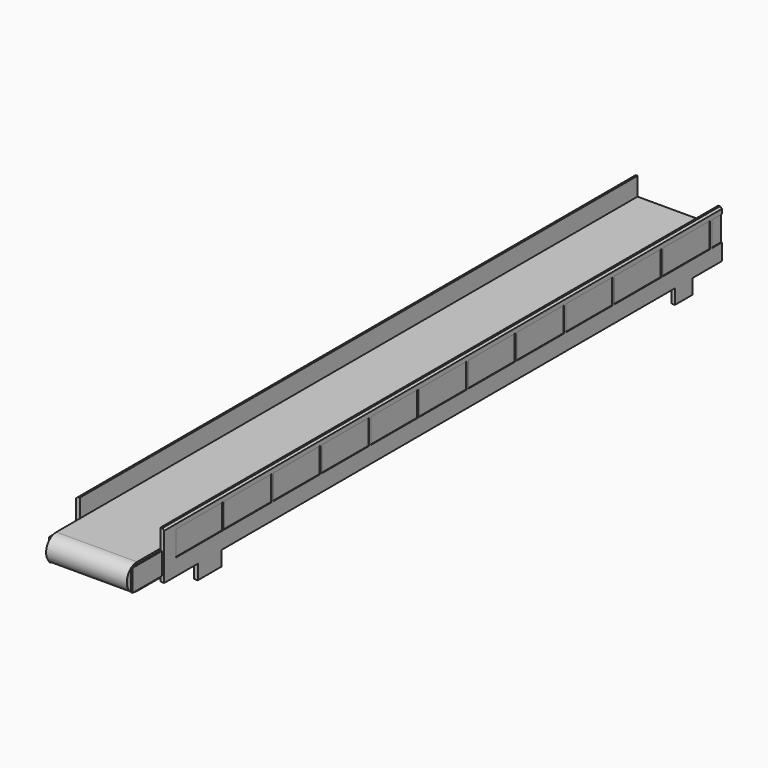
from build123d import *

# Parameters (mm, degrees)
F1_R          = 150
F2_DEPTH      = 1100
F4_DEPTH      = 1100
F6_START      = -400
F6_DEPTH      = 12000
F7_W          = 20
F7_H          = 300
F8_DEPTH      = 500
F8_DEPTH_BACK = 12500
F9_W          = 800
F9_H          = 340
F10_DEPTH     = 10
F11_W         = 800
F11_H         = 340
F12_DEPTH     = 10
F13_W         = 50
F13_H         = 400
F14_DEPTH     = 200
F15_W         = 1814.6319389343
F15_H         = 1127.1775364876
F16_DEPTH     = 3000
F17_W         = 50
F17_H         = 300
F18_DEPTH     = 200


with BuildPart() as f2:
    # F1 (on Right) → F2 (new body)
    with BuildSketch(Plane.YZ):
        Circle(F1_R)
    extrude(amount=F2_DEPTH)


with BuildPart() as f2b:
    # F1 (on Right) → F2, piece 2 (new body)
    with BuildSketch(Plane.YZ):
        with Locations((12700, 0)):
            Circle(F1_R)
    extrude(amount=F2_DEPTH)


with BuildPart() as f4:
    # F3 (on face) → F4 (new body)
    with BuildSketch(Plane.YZ.offset(1100)):
        with BuildLine():
            ThreePointArc((0, -175), (123.7436867076, -123.7436867076), (175, 0))
            ThreePointArc((175, 0), (123.7436867076, 123.7436867076), (0, 175))
            Line((0, 175), (0, -175))
        make_face()
        with BuildLine():
            ThreePointArc((0, 175), (123.7436867076, 123.7436867076), (175, 0))
            ThreePointArc((175, 0), (123.7436867076, -123.7436867076), (0, -175))
            Line((0, -175), (12700, -175))
            ThreePointArc((12700, -175), (12525, 0), (12700, 175))
            Line((12700, 175), (0, 175))
        make_face()
        with BuildLine():
            Line((0, -175), (0, 175))
            ThreePointArc((0, 175), (-175, 0), (0, -175))
        make_face()
        with BuildLine():
            Line((12700, -175), (12700, 175))
            ThreePointArc((12700, 175), (12525, 0), (12700, -175))
        make_face()
        with BuildLine():
            ThreePointArc((12875, 0), (12823.7436867076, 123.7436867076), (12700, 175))
            Line((12700, 175), (12700, -175))
            ThreePointArc((12700, -175), (12823.7436867076, -123.7436867076), (12875, 0))
        make_face()
    extrude(amount=-F4_DEPTH)


with BuildPart() as f6:
    # F5 (on Front) → F6 (new body)
    with BuildSketch(Plane.XZ.offset(F6_START)):
        Polygon((0, -225), (0, 425), (-25, 425), (-50, 401.8485546112), (-50, -225), align=None)
    extrude(amount=-F6_DEPTH)

    # F7 (on face) → F8 (join, two sides)
    with BuildSketch(Plane.XZ.offset(-400)) as f8_sk:
        with Locations((-10, 0)):
            Rectangle(F7_W, F7_H)
    extrude(amount=F8_DEPTH)
    extrude(f8_sk.sketch, amount=-F8_DEPTH_BACK)

    # F9 (on face) → F10 (cut)
    with BuildSketch(Plane(origin=(-50, 0, 0), x_dir=(0, -1, 0), z_dir=(-1, 0, 0))):
        with Locations((-1000, 170)):
            Rectangle(F9_W, F9_H)
        with Locations((-1830, 170)):
            Rectangle(F9_W, F9_H)
        with Locations((-2660, 170)):
            Rectangle(F9_W, F9_H)
        with Locations((-3490, 170)):
            Rectangle(F9_W, F9_H)
        with Locations((-4320, 170)):
            Rectangle(F9_W, F9_H)
        with Locations((-5150, 170)):
            Rectangle(F9_W, F9_H)
        with Locations((-5980, 170)):
            Rectangle(F9_W, F9_H)
        with Locations((-6810, 170)):
            Rectangle(F9_W, F9_H)
        with Locations((-7640, 170)):
            Rectangle(F9_W, F9_H)
        with Locations((-8470, 170)):
            Rectangle(F9_W, F9_H)
        with Locations((-9300, 170)):
            Rectangle(F9_W, F9_H)
        with Locations((-10130, 170)):
            Rectangle(F9_W, F9_H)
        with Locations((-10960, 170)):
            Rectangle(F9_W, F9_H)
        with Locations((-11790, 170)):
            Rectangle(F9_W, F9_H)
    extrude(amount=-F10_DEPTH, mode=Mode.SUBTRACT)

    # F13 (on face) → F14, piece 2 (join)
    with BuildSketch(Plane(origin=(0, 0, -225), x_dir=(1, 0, 0), z_dir=(0, 0, -1))):
        with Locations((-25, -1171.534705162)):
            Rectangle(F13_W, F13_H)
        with Locations((-25, -11671.534705162)):
            Rectangle(F13_W, F13_H)
    extrude(amount=F14_DEPTH)


with BuildPart() as f6b:
    # F5 (on Front) → F6, piece 2 (new body)
    with BuildSketch(Plane.XZ.offset(F6_START)):
        Polygon((1125, 425), (1100, 425), (1100, -225), (1150, -225), (1150, 401.8485546112), align=None)
    extrude(amount=-F6_DEPTH)

    # F7 (on face) → F8, piece 2 (join, two sides)
    with BuildSketch(Plane.XZ.offset(-400)) as f8_2_sk:
        with Locations((1110, 0)):
            Rectangle(F7_W, F7_H)
    extrude(amount=F8_DEPTH)
    extrude(f8_2_sk.sketch, amount=-F8_DEPTH_BACK)

    # F11 (on face) → F12 (cut)
    with BuildSketch(Plane.YZ.offset(1150)):
        with Locations((1000, 170)):
            Rectangle(F11_W, F11_H)
        with Locations((1830, 170)):
            Rectangle(F11_W, F11_H)
        with Locations((2660, 170)):
            Rectangle(F11_W, F11_H)
        with Locations((3490, 170)):
            Rectangle(F11_W, F11_H)
        with Locations((4320, 170)):
            Rectangle(F11_W, F11_H)
        with Locations((5150, 170)):
            Rectangle(F11_W, F11_H)
        with Locations((5980, 170)):
            Rectangle(F11_W, F11_H)
        with Locations((6810, 170)):
            Rectangle(F11_W, F11_H)
        with Locations((7640, 170)):
            Rectangle(F11_W, F11_H)
        with Locations((8470, 170)):
            Rectangle(F11_W, F11_H)
        with Locations((9300, 170)):
            Rectangle(F11_W, F11_H)
        with Locations((10130, 170)):
            Rectangle(F11_W, F11_H)
        with Locations((10960, 170)):
            Rectangle(F11_W, F11_H)
        with Locations((11790, 170)):
            Rectangle(F11_W, F11_H)
    extrude(amount=-F12_DEPTH, mode=Mode.SUBTRACT)

    # F13 (on face) → F14 (join)
    with BuildSketch(Plane(origin=(0, 0, -225), x_dir=(1, 0, 0), z_dir=(0, 0, -1))):
        with Locations((1125, -1171.534705162)):
            Rectangle(F13_W, F13_H)
        with Locations((1125, -11671.534705162)):
            Rectangle(F13_W, F13_H)
    extrude(amount=F14_DEPTH)


with BuildPart() as f16_tool:
    # F15 (on face) → F16 (new body)
    with BuildSketch(Plane(origin=(0, 12900, 0), x_dir=(-1, 0, 0), z_dir=(0, 1, 0))):
        with Locations((-568.1853294373, 30.6665599346)):
            Rectangle(F15_W, F15_H)
    extrude(amount=-F16_DEPTH)


with BuildPart() as f2b_1:
    add(f2b.part)

    # F16: cut by f16_tool
    add(f16_tool.part, mode=Mode.SUBTRACT)


with BuildPart() as f4_1:
    add(f4.part)

    # F16: cut by f16_tool
    add(f16_tool.part, mode=Mode.SUBTRACT)


with BuildPart() as f6_1:
    add(f6.part)

    # F16: cut by f16_tool
    add(f16_tool.part, mode=Mode.SUBTRACT)

    # F17 (on face) → F18, piece 2 (join)
    with BuildSketch(Plane(origin=(0, 0, -225), x_dir=(1, 0, 0), z_dir=(0, 0, -1))):
        with Locations((-25, -9250)):
            Rectangle(F17_W, F17_H)
    extrude(amount=F18_DEPTH)


with BuildPart() as f6b_1:
    add(f6b.part)

    # F16: cut by f16_tool
    add(f16_tool.part, mode=Mode.SUBTRACT)

    # F17 (on face) → F18 (join)
    with BuildSketch(Plane(origin=(0, 0, -225), x_dir=(1, 0, 0), z_dir=(0, 0, -1))):
        with Locations((1125, -9250)):
            Rectangle(F17_W, F17_H)
    extrude(amount=F18_DEPTH)


solid = Compound([f2.part, f4_1.part, f6_1.part, f6b_1.part])
